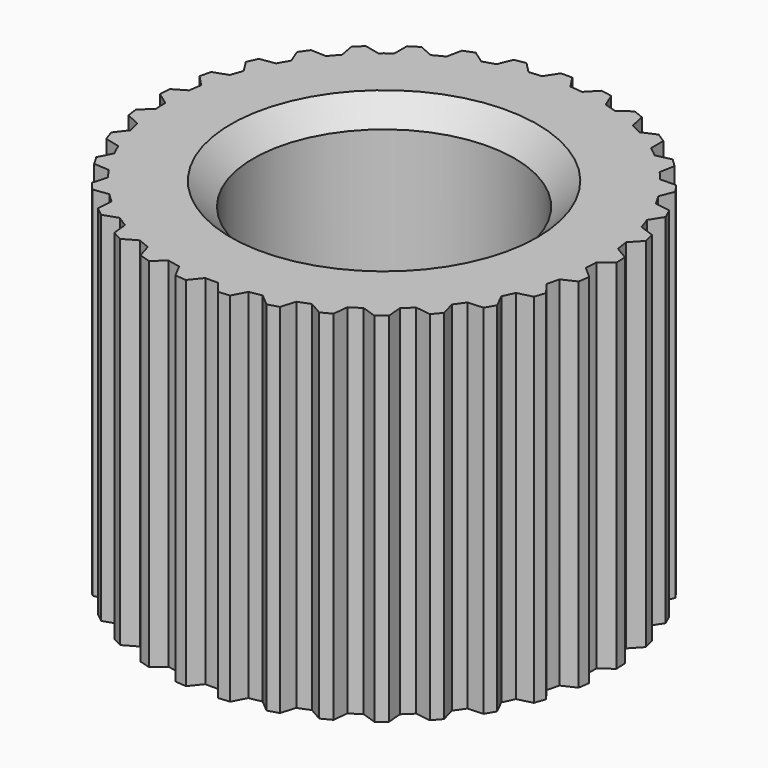
from build123d import *

# Parameters (mm, degrees)
F0_R            = 2.921
F1_DEPTH        = 8.001
F2_DEPTH        = 8.001
F2_COPIES_COUNT = 33
F3_SIZE         = 0.508


# Not quite as in the source:
# - a pattern or mirror of a feature is missing from the dataset's text; its kind, count and spacing are read off the source's solid


with BuildPart() as f1:
    # F0 (on Top) → F1 (new body)
    with BuildSketch(Plane.XY):
        with BuildLine():
            ThreePointArc((-0.3175, 4.8155445954), (-3.298334504, -3.5229626027), (4.826, 0))
            ThreePointArc((4.826, 0), (3.5229626027, 3.298334504), (0.3175, 4.8155445954))
            ThreePointArc((0.3175, 4.8155445954), (0, 4.826), (-0.3175, 4.8155445954))
        make_face()
        Circle(F0_R, mode=Mode.SUBTRACT)
    extrude(amount=F1_DEPTH)

    # F0 (on Top) → F2 (join, through all)
    with BuildSketch(Plane.XY):
        with BuildLine():
            ThreePointArc((-0.3175, 4.8155445954), (0, 4.826), (0.3175, 4.8155445954))
            Line((0.3175, 4.8155445954), (0.127, 5.1054))
            Line((0.127, 5.1054), (-0.127, 5.1054))
            Line((-0.127, 5.1054), (-0.3175, 4.8155445954))
        make_face()
    f2 = extrude(amount=F2_DEPTH)

    # F2_copies: F2 ×33 about axis
    f2_copies_axis = Axis((0, 0, 0), (0, 0, 1))
    for i in range(1, F2_COPIES_COUNT):
        add(f2.rotate(f2_copies_axis, i * 360 / F2_COPIES_COUNT))

    # F3
    f3_edges = [f1.edges().sort_by_distance(p)[0] for p in [
        (-2.921, 0, 8.001),
    ]]
    chamfer(f3_edges, length=F3_SIZE)


solid = f1.part
